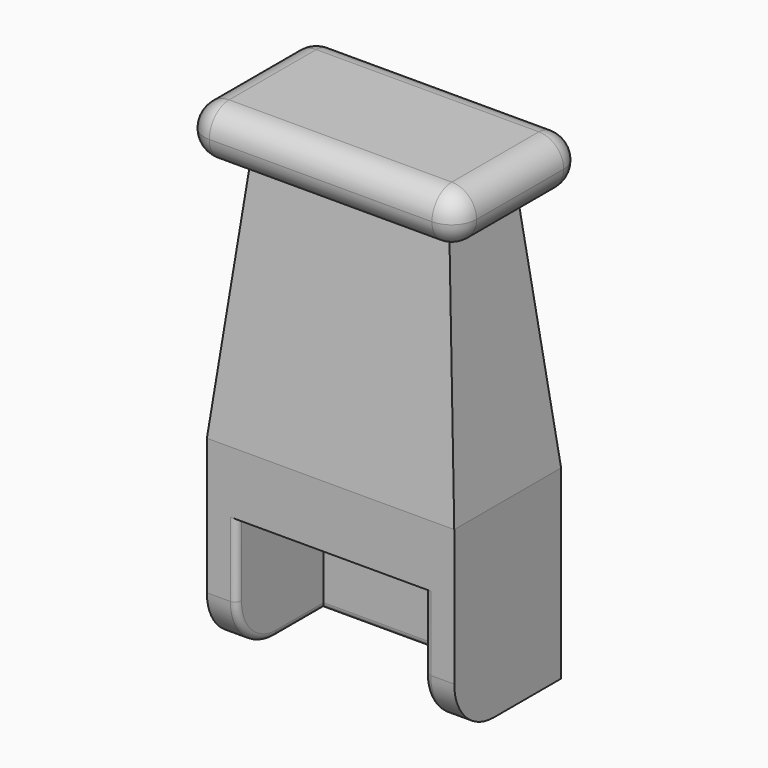
from build123d import *

# Parameters (mm, degrees)
F0_W     = 1.2
F0_H     = 4.4
F0_W_2   = 7.6
F0_R     = 0.55
F1_DEPTH = 12.5
F2_DEPTH = 5
F3_DEPTH = 1.5
F4_DEPTH = 5
F5_R     = 2
F6_R     = 0.25
F7_SIZE2 = 10
F7_SIZE  = 1
F8_W     = 11.0000001401
F8_H     = 6.4000001401
F8_W_2   = 8
F8_H_2   = 3.4
F9_DEPTH = 2
F10_R    = 0.99999


# Not quite as in the source:
# - a fillet or chamfer is up to 0.001 mm smaller than in the source, because OpenCascade refuses the exact size


with BuildPart() as f1:
    # F0 (on Top) → F1 (new body)
    with BuildSketch(Plane.XY):
        Polygon((-5, 2.2), (-3.8, 2.2), (3.8, 2.2), (5, 2.2), (5, 3.2), (-5, 3.2), align=None)
        with Locations((-4.4, 0)):
            Rectangle(F0_W, F0_H)
        Rectangle(F0_W_2, F0_H)
        with BuildLine():
            Line((2.05, 1.05), (2.05, 0))
            Line((2.05, 0), (2.05, -1.05))
            ThreePointArc((2.05, -1.05), (2.2267766953, -1.4767766953), (1.8, -1.3))
            Line((1.8, -1.3), (-1.8, -1.3))
            ThreePointArc((-1.8, -1.3), (-2.2267766953, -1.4767766953), (-2.05, -1.05))
            Line((-2.05, -1.05), (-2.05, 0))
            Line((-2.05, 0), (-2.05, 1.05))
            ThreePointArc((-2.05, 1.05), (-2.2267766953, 1.4767766953), (-1.8, 1.3))
            Line((-1.8, 1.3), (1.8, 1.3))
            ThreePointArc((1.8, 1.3), (2.2267766953, 1.4767766953), (2.05, 1.05))
        make_face(mode=Mode.SUBTRACT)
        with Locations((4.4, 0)):
            Rectangle(F0_W, F0_H)
        with BuildLine():
            ThreePointArc((0, 0.3201562119), (1.1620185175, 1.0374246961), (2.05, 0))
            Line((2.05, 0), (2.05, 1.05))
            ThreePointArc((2.05, 1.05), (2.2267766953, 1.4767766953), (1.8, 1.3))
            Line((1.8, 1.3), (-1.8, 1.3))
            ThreePointArc((-1.8, 1.3), (-2.2267766953, 1.4767766953), (-2.05, 1.05))
            Line((-2.05, 1.05), (-2.05, 0))
            ThreePointArc((-2.05, 0), (-1.1620185175, 1.0374246961), (0, 0.3201562119))
        make_face()
        with BuildLine():
            Line((2.05, -1.05), (2.05, 0))
            ThreePointArc((2.05, 0), (1.1620185175, -1.0374246961), (0, -0.3201562119))
            ThreePointArc((0, -0.3201562119), (-1.1620185175, -1.0374246961), (-2.05, 0))
            Line((-2.05, 0), (-2.05, -1.05))
            ThreePointArc((-2.05, -1.05), (-2.2267766953, -1.4767766953), (-1.8, -1.3))
            Line((-1.8, -1.3), (1.8, -1.3))
            ThreePointArc((1.8, -1.3), (2.2267766953, -1.4767766953), (2.05, -1.05))
        make_face()
        with BuildLine():
            ThreePointArc((0, -0.3201562119), (-0.05, 0), (0, 0.3201562119))
            ThreePointArc((0, 0.3201562119), (-1.1620185175, 1.0374246961), (-2.05, 0))
            ThreePointArc((-2.05, 0), (-1.1620185175, -1.0374246961), (0, -0.3201562119))
        make_face()
        with Locations((-1, 0)):
            Circle(F0_R, mode=Mode.SUBTRACT)
        with BuildLine():
            ThreePointArc((0, -0.3201562119), (1.1620185175, -1.0374246961), (2.05, 0))
            ThreePointArc((2.05, 0), (1.1620185175, 1.0374246961), (0, 0.3201562119))
            ThreePointArc((0, 0.3201562119), (0.0374246961, 0.1620185175), (0.05, 0))
            ThreePointArc((0.05, 0), (0.0374246961, -0.1620185175), (0, -0.3201562119))
        make_face()
        with Locations((1, 0)):
            Circle(F0_R, mode=Mode.SUBTRACT)
        with Locations((-1, 0)):
            Circle(F0_R)
        with Locations((1, 0)):
            Circle(F0_R)
        with BuildLine():
            ThreePointArc((0.05, 0), (0.0374246961, 0.1620185175), (0, 0.3201562119))
            ThreePointArc((0, 0.3201562119), (-0.05, 0), (0, -0.3201562119))
            ThreePointArc((0, -0.3201562119), (0.0374246961, -0.1620185175), (0.05, 0))
        make_face()
    extrude(amount=F1_DEPTH)

    # F0 (on Top) → F2 (join)
    with BuildSketch(Plane.XY):
        with Locations((-4.4, 0)):
            Rectangle(F0_W, F0_H)
        with Locations((4.4, 0)):
            Rectangle(F0_W, F0_H)
        Polygon((-5, 2.2), (-3.8, 2.2), (3.8, 2.2), (5, 2.2), (5, 3.2), (-5, 3.2), align=None)
    extrude(amount=-F2_DEPTH)

    # F0 (on Top) → F3 (cut)
    with BuildSketch(Plane.XY):
        with BuildLine():
            ThreePointArc((0, -0.3201562119), (-0.05, 0), (0, 0.3201562119))
            ThreePointArc((0, 0.3201562119), (-1.1620185175, 1.0374246961), (-2.05, 0))
            ThreePointArc((-2.05, 0), (-1.1620185175, -1.0374246961), (0, -0.3201562119))
        make_face()
        with Locations((-1, 0)):
            Circle(F0_R, mode=Mode.SUBTRACT)
        with BuildLine():
            ThreePointArc((0, -0.3201562119), (1.1620185175, -1.0374246961), (2.05, 0))
            ThreePointArc((2.05, 0), (1.1620185175, 1.0374246961), (0, 0.3201562119))
            ThreePointArc((0, 0.3201562119), (0.0374246961, 0.1620185175), (0.05, 0))
            ThreePointArc((0.05, 0), (0.0374246961, -0.1620185175), (0, -0.3201562119))
        make_face()
        with Locations((1, 0)):
            Circle(F0_R, mode=Mode.SUBTRACT)
        with BuildLine():
            ThreePointArc((0.05, 0), (0.0374246961, 0.1620185175), (0, 0.3201562119))
            ThreePointArc((0, 0.3201562119), (-0.05, 0), (0, -0.3201562119))
            ThreePointArc((0, -0.3201562119), (0.0374246961, -0.1620185175), (0.05, 0))
        make_face()
    extrude(amount=F3_DEPTH, mode=Mode.SUBTRACT)

    # F0 (on Top) → F4 (cut)
    with BuildSketch(Plane.XY):
        with Locations((-1, 0)):
            Circle(F0_R)
        with Locations((1, 0)):
            Circle(F0_R)
    extrude(amount=F4_DEPTH, mode=Mode.SUBTRACT)

    # F5
    f5_edges = [f1.edges().sort_by_distance(p)[0] for p in [
        (4.4, -2.2, -5),
        (-4.4, -2.2, -5),
    ]]
    fillet(f5_edges, radius=F5_R)

    # F6
    f6_edges = [f1.edges().sort_by_distance(p)[0] for p in [
        (0.45, 0, 1.5),
        (2.05, 0, 0),
        (-1.55, 0, 1.5),
        (-2.05, 0, 0),
        (-3.8, 1, -5),
        (0, 2.2, -5),
        (3.8, 1, -5),
        (-3.8, -2.2, -1.5),
        (3.8, -2.2, -1.5),
    ]]
    fillet(f6_edges, radius=F6_R)

    # F7
    f7_edges = [f1.edges().sort_by_distance(p)[0] for p in [
        (0, -2.2, 12.5),
        (-5, 0.5, 12.5),
        (5, 0.5, 12.5),
        (0, 3.2, 12.5),
    ]]
    f7_side = f1.faces().sort_by_distance((0, 0.5, 12.5))[0]
    chamfer(f7_edges, length=F7_SIZE, length2=F7_SIZE2, reference=f7_side)

    # F8 (on face) → F9 (join)
    with BuildSketch(Plane.XY.offset(12.5)):
        with Locations((0, 0.5)):
            Rectangle(F8_W, F8_H)
        with Locations((0, 0.5)):
            Rectangle(F8_W_2, F8_H_2, mode=Mode.SUBTRACT)
        with Locations((0, 0.5)):
            Rectangle(F8_W_2, F8_H_2)
    extrude(amount=F9_DEPTH)

    # F10 (radius 1 in the source; OpenCascade refuses exactly that, so slightly less here)
    f10_edges = [f1.edges().sort_by_distance(p)[0] for p in [
        (5.5, -2.7, 13.5),
        (-5.5, -2.7, 13.5),
        (5.5, 3.7, 13.5),
        (-5.5, 3.7, 13.5),
        (0, 3.7, 12.5),
        (0, 3.7, 14.5),
        (-5.5, 0.5, 14.5),
        (5.5, 0.5, 14.5),
        (0, -2.7, 14.5),
        (5.5, 0.5, 12.5),
        (0, -2.7, 12.5),
        (-5.5, 0.5, 12.5),
    ]]
    fillet(f10_edges, radius=F10_R)


solid = f1.part
